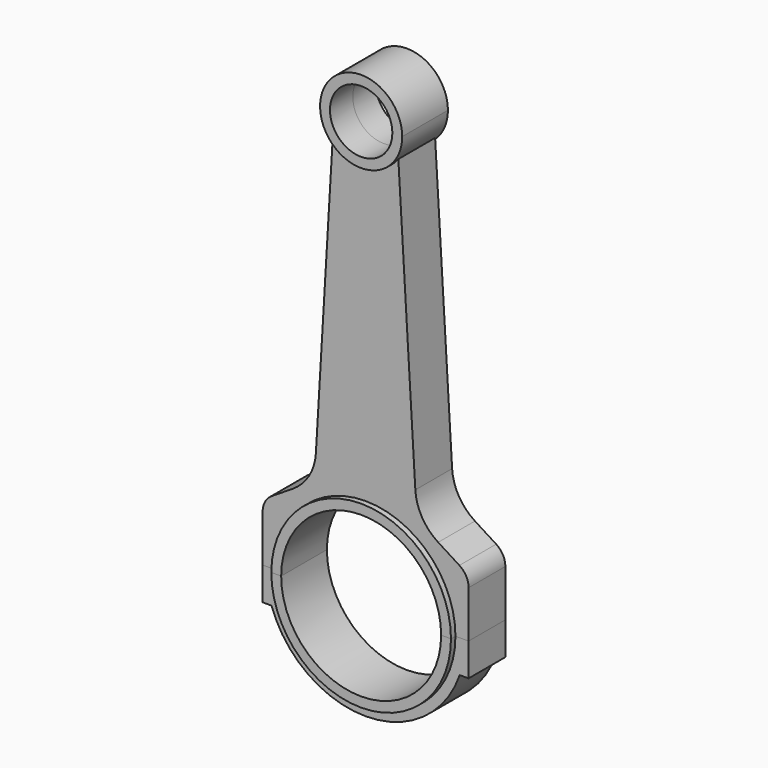
from build123d import *

# Parameters (mm, degrees)
F1_DEPTH = 11.049
F2_DEPTH = 8.89
F0_R     = 12.065
F3_DEPTH = 11.049
F4_DEPTH = 11.049
F5_DEPTH = 8.89


with BuildPart() as f1:
    # F0 (on Front) → F1 (new body, symmetric)
    with BuildSketch(Plane.XZ):
        with BuildLine():
            ThreePointArc((-30.9245, 0), (0, 30.9245), (30.9245, 0))
            Line((30.9245, 0), (34.7345, 0))
            ThreePointArc((34.7345, 0), (0, 34.7345), (-34.7345, 0))
            Line((-34.7345, 0), (-30.9245, 0))
        make_face()
    extrude(amount=F1_DEPTH, both=True)

    # F0 (on Front) → F2 (join, symmetric)
    with BuildSketch(Plane.XZ):
        with BuildLine():
            ThreePointArc((-34.7345, 0), (0, 34.7345), (34.7345, 0))
            Line((34.7345, 0), (39.8145, 0))
            Line((39.8145, 0), (39.8145, 18.174736774))
            ThreePointArc((39.8145, 18.174736774), (38.8693796529, 21.8503838762), (36.2684680788, 24.6142386253))
            Line((36.2684680788, 24.6142386253), (28.0604028001, 29.8070930892))
            ThreePointArc((28.0604028001, 29.8070930892), (21.8384993627, 36.2250090023), (19.2289533596, 44.7743947528))
            Line((19.2289533596, 44.7743947528), (12.6564985929, 155.2378723942))
            ThreePointArc((12.6564985929, 155.2378723942), (0, 148.9456), (-12.6564985929, 155.2378723942))
            Line((-12.6564985929, 155.2378723942), (-19.2289533596, 44.7743947528))
            ThreePointArc((-19.2289533596, 44.7743947528), (-21.8384993627, 36.2250090023), (-28.0604028001, 29.8070930892))
            Line((-28.0604028001, 29.8070930892), (-36.2684680788, 24.6142386253))
            ThreePointArc((-36.2684680788, 24.6142386253), (-38.8693796529, 21.8503838762), (-39.8145, 18.174736774))
            Line((-39.8145, 18.174736774), (-39.8145, 0))
            Line((-39.8145, 0), (-34.7345, 0))
        make_face()
    extrude(amount=F2_DEPTH, both=True)

    # F0 (on Front) → F3 (join, symmetric)
    with BuildSketch(Plane.XZ):
        with BuildLine():
            ThreePointArc((-12.6564985929, 155.2378723942), (0, 148.9456), (12.6564985929, 155.2378723942))
            ThreePointArc((12.6564985929, 155.2378723942), (15.048879363, 159.7662103318), (15.875, 164.8206))
            ThreePointArc((15.875, 164.8206), (-5.0543896682, 179.869479363), (-12.6564985929, 155.2378723942))
        make_face()
        with Locations((0, 164.8206)):
            Circle(F0_R, mode=Mode.SUBTRACT)
    extrude(amount=F3_DEPTH, both=True)


with BuildPart() as f4:
    # F0 (on Front) → F4 (new body, symmetric)
    with BuildSketch(Plane.XZ):
        with BuildLine():
            Line((34.7345, 0), (30.9245, 0))
            ThreePointArc((30.9245, 0), (0, -30.9245), (-30.9245, 0))
            Line((-30.9245, 0), (-34.7345, 0))
            ThreePointArc((-34.7345, 0), (0, -34.7345), (34.7345, 0))
        make_face()
    extrude(amount=F4_DEPTH, both=True)

    # F0 (on Front) → F5 (join, symmetric)
    with BuildSketch(Plane.XZ):
        with BuildLine():
            Line((39.8145, 0), (34.7345, 0))
            ThreePointArc((34.7345, 0), (0, -34.7345), (-34.7345, 0))
            Line((-34.7345, 0), (-39.8145, 0))
            Line((-39.8145, 0), (-39.8145, -12.7))
            Line((-39.8145, -12.7), (-36.3921486072, -12.7))
            ThreePointArc((-36.3921486072, -12.7), (0, -38.5445), (36.3921486072, -12.7))
            Line((36.3921486072, -12.7), (39.8145, -12.7))
            Line((39.8145, -12.7), (39.8145, 0))
        make_face()
    extrude(amount=F5_DEPTH, both=True)


solid = Compound([f1.part, f4.part])
